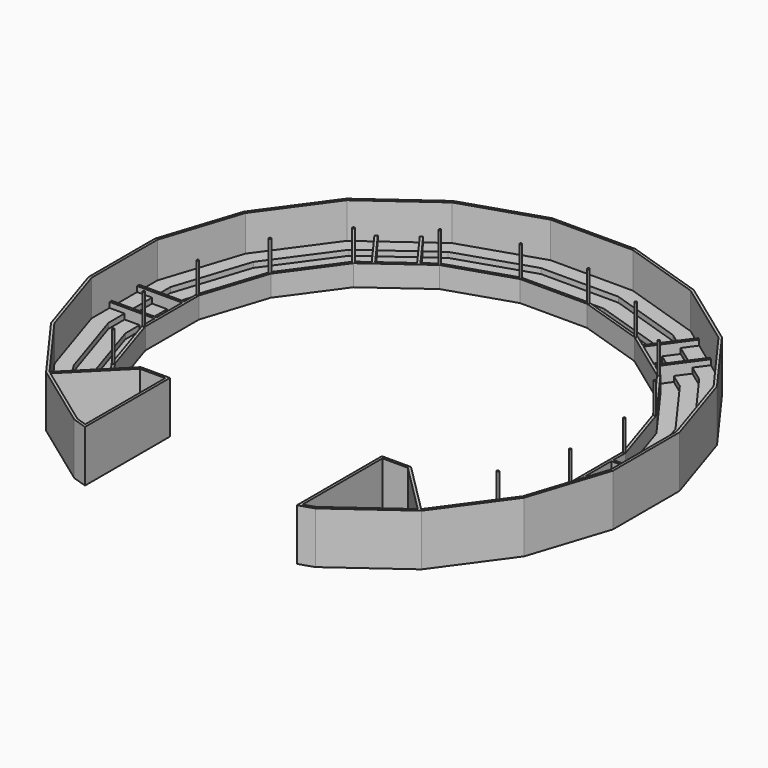
from build123d import *

# Parameters (mm, degrees)
F1_DEPTH = 2971.8
F2_DEPTH = 304.8
F0_W     = 863.6
F0_H     = 1828.8
F3_DEPTH = 609.6
F4_DEPTH = 914.4
F0_R     = 60.96
F5_DEPTH = 1219.2
F6_DEPTH = 2971.8


with BuildPart() as f1:
    # F0 (on Top) → F1 (new body)
    with BuildSketch(Plane.XY):
        Polygon((2389.6410818405, 15087.6), (-2389.6410818405, 15087.6), (-6935.0085268224, 13610.7205905095), (-8128.5036328315, 12743.5956390277), (-9655.127382741, 11634.4385604554), (-10801.5290181534, 10801.5290181534), (-13610.7205905095, 6935.0085268224), (-15087.6, 2389.6410818405), (-15087.6, 914.4), (-15087.6, 0), (-15087.6, -2389.6410818405), (-13610.7205905095, -6935.0085268224), (-10801.5290181534, -10801.5290181534), (-6935.0085268224, -13610.7205905095), (-6096, -13883.3309861815), (-6096, -7924.8), (-6096, -7772.4), (-7772.4, -7772.4), (-8728.5082974977, -8728.5082974977), (-8837.6146512164, -8837.6146512164), (-9455.8839889558, -9455.8839889558), (-10074.1533266953, -10074.1533266953), (-10692.4226644347, -10692.4226644347), (-13473.2385643428, -6864.9579356424), (-14935.2, -2365.503293135), (-14935.2, -1066.8), (-14935.2, -914.4), (-14935.2, 914.4), (-14935.2, 1066.8), (-14935.2, 2365.503293135), (-13473.2385643428, 6864.9579356424), (-10692.4226644347, 10692.4226644347), (-9688.8431002343, 11421.5658980633), (-9565.5489102916, 11511.1443705127), (-8038.9251603821, 12620.301449085), (-7915.6309704393, 12709.8799215343), (-6864.9579356424, 13473.2385643428), (-2365.503293135, 14935.2), (2365.503293135, 14935.2), (6864.9579356424, 13473.2385643428), (7915.6309704393, 12709.8799215343), (8038.9251603821, 12620.301449085), (9518.455439695, 11545.3597796925), (9641.7496296377, 11455.7813072431), (10692.4226644347, 10692.4226644347), (13473.2385643428, 6864.9579356424), (14935.2, 2365.503293135), (14935.2, 1066.8), (14935.2, 914.4), (14935.2, -914.4), (14935.2, -1066.8), (14935.2, -2365.503293135), (13473.2385643428, -6864.9579356424), (10692.4226644347, -10692.4226644347), (10074.1533266953, -10074.1533266953), (9455.8839889558, -9455.8839889558), (8837.6146512164, -8837.6146512164), (8728.5082974977, -8728.5082974977), (7772.4, -7772.4), (6705.6, -7772.4), (6096, -7772.4), (6096, -13883.3309861815), (6935.0085268224, -13610.7205905095), (10801.5290181534, -10801.5290181534), (13610.7205905095, -6935.0085268224), (15087.6, -2389.6410818405), (15087.6, -914.4), (15087.6, 914.4), (15087.6, 2389.6410818405), (13610.7205905095, 6935.0085268224), (10801.5290181534, 10801.5290181534), (6935.0085268224, 13610.7205905095), align=None)
        Polygon((-6864.9579356424, -13473.2385643428), (-10567.5915969054, -10783.117743811), (-7709.2738530943, -7924.8), (-6248.4, -7924.8), (-6248.4, -13673.5703815017), align=None, mode=Mode.SUBTRACT)
        Polygon((7709.2738530943, -7924.8), (10567.5915969054, -10783.117743811), (6864.9579356424, -13473.2385643428), (6248.4, -13673.5703815017), (6248.4, -7924.8), align=None, mode=Mode.SUBTRACT)
    extrude(amount=F1_DEPTH)


with BuildPart() as f2:
    # F0 (on Top) → F2 (new body)
    with BuildSketch(Plane.XY):
        Polygon((-9455.8839889558, -9455.8839889558), (-8837.6146512164, -8837.6146512164), (-11136.0441195078, -5674.097885582), (-12344.4, -1955.1608851422), (-12344.4, -1066.8), (-13208, -1066.8), (-13208, -2091.9416878065), (-11915.1089344528, -6071.0512356021), align=None)
    extrude(amount=F2_DEPTH)

    # F0 (on Top) → F3, piece 2 (join)
    with BuildSketch(Plane.XY):
        Polygon((-10074.1533266953, -10074.1533266953), (-9455.8839889558, -9455.8839889558), (-11915.1089344528, -6071.0512356021), (-13208, -2091.9416878065), (-13208, -1066.8), (-14071.6, -1066.8), (-14071.6, -2228.7224904707), (-12694.1737493978, -6468.0045856223), align=None)
    extrude(amount=F3_DEPTH)

    # F0 (on Top) → F4 (join)
    with BuildSketch(Plane.XY):
        Polygon((-10692.4226644347, -10692.4226644347), (-10074.1533266953, -10074.1533266953), (-12694.1737493978, -6468.0045856223), (-14071.6, -2228.7224904707), (-14071.6, -1066.8), (-14935.2, -1066.8), (-14935.2, -2365.503293135), (-13473.2385643428, -6864.9579356424), align=None)
    extrude(amount=F4_DEPTH)



with BuildPart() as f2b:
    # F0 (on Top) → F2, piece 2 (new body)
    with BuildSketch(Plane.XY):
        Polygon((-13208, 2091.9416878065), (-13208, 1066.8), (-12344.4, 1066.8), (-12344.4, 1955.1608851422), (-11136.0441195078, 5674.097885582), (-8837.6146512164, 8837.6146512164), (-8166.009068595, 9325.5646690367), (-8673.6204124748, 10024.2317453789), (-9455.8839889558, 9455.8839889558), (-11915.1089344528, 6071.0512356021), align=None)
    extrude(amount=F2_DEPTH)

    # F0 (on Top) → F3 (join)
    with BuildSketch(Plane.XY):
        Polygon((-14071.6, 2228.7224904707), (-14071.6, 1066.8), (-13208, 1066.8), (-13208, 2091.9416878065), (-11915.1089344528, 6071.0512356021), (-9455.8839889558, 9455.8839889558), (-8673.6204124748, 10024.2317453789), (-9181.2317563546, 10722.8988217211), (-10074.1533266953, 10074.1533266953), (-12694.1737493978, 6468.0045856223), align=None)
    extrude(amount=F3_DEPTH)

    # F0 (on Top) → F4, piece 2 (join)
    with BuildSketch(Plane.XY):
        Polygon((-14935.2, 2365.503293135), (-14935.2, 1066.8), (-14071.6, 1066.8), (-14071.6, 2228.7224904707), (-12694.1737493978, 6468.0045856223), (-10074.1533266953, 10074.1533266953), (-9181.2317563546, 10722.8988217211), (-9688.8431002343, 11421.5658980633), (-10692.4226644347, 10692.4226644347), (-13473.2385643428, 6864.9579356424), align=None)
    extrude(amount=F4_DEPTH)


with BuildPart() as f2c:
    # F0 (on Top) → F2, piece 3 (new body)
    with BuildSketch(Plane.XY):
        Polygon((11136.0441195078, -5674.097885582), (8837.6146512164, -8837.6146512164), (9455.8839889558, -9455.8839889558), (11915.1089344528, -6071.0512356021), (13208, -2091.9416878065), (13208, -1066.8), (12344.4, -1066.8), (12344.4, -1955.1608851422), align=None)
    extrude(amount=F2_DEPTH)

    # F0 (on Top) → F3, piece 5 (join)
    with BuildSketch(Plane.XY):
        Polygon((11915.1089344528, -6071.0512356021), (9455.8839889558, -9455.8839889558), (10074.1533266953, -10074.1533266953), (12694.1737493978, -6468.0045856223), (14071.6, -2228.7224904707), (14071.6, -1066.8), (13208, -1066.8), (13208, -2091.9416878065), align=None)
    extrude(amount=F3_DEPTH)

    # F0 (on Top) → F4, piece 5 (join)
    with BuildSketch(Plane.XY):
        Polygon((12694.1737493978, -6468.0045856223), (10074.1533266953, -10074.1533266953), (10692.4226644347, -10692.4226644347), (13473.2385643428, -6864.9579356424), (14935.2, -2365.503293135), (14935.2, -1066.8), (14071.6, -1066.8), (14071.6, -2228.7224904707), align=None)
    extrude(amount=F4_DEPTH)


with BuildPart() as f2d:
    # F0 (on Top) → F2, piece 4 (new body)
    with BuildSketch(Plane.XY):
        Polygon((12344.4, 1066.8), (13208, 1066.8), (13208, 2091.9416878065), (11915.1089344528, 6071.0512356021), (9455.8839889558, 9455.8839889558), (8626.5269418782, 10058.4471545587), (8118.9155979984, 9359.7800782165), (8837.6146512164, 8837.6146512164), (11136.0441195078, 5674.097885582), (12344.4, 1955.1608851422), align=None)
    extrude(amount=F2_DEPTH)

    # F0 (on Top) → F3, piece 4 (join)
    with BuildSketch(Plane.XY):
        Polygon((13208, 1066.8), (14071.6, 1066.8), (14071.6, 2228.7224904707), (12694.1737493978, 6468.0045856223), (10074.1533266953, 10074.1533266953), (9134.1382857579, 10757.1142309009), (8626.5269418782, 10058.4471545587), (9455.8839889558, 9455.8839889558), (11915.1089344528, 6071.0512356021), (13208, 2091.9416878065), align=None)
    extrude(amount=F3_DEPTH)

    # F0 (on Top) → F4, piece 4 (join)
    with BuildSketch(Plane.XY):
        Polygon((14071.6, 1066.8), (14935.2, 1066.8), (14935.2, 2365.503293135), (13473.2385643428, 6864.9579356424), (10692.4226644347, 10692.4226644347), (9641.7496296377, 11455.7813072431), (9134.1382857579, 10757.1142309009), (10074.1533266953, 10074.1533266953), (12694.1737493978, 6468.0045856223), (14071.6, 2228.7224904707), align=None)
    extrude(amount=F4_DEPTH)


with BuildPart() as f2e:
    # F0 (on Top) → F2, piece 5 (new body)
    with BuildSketch(Plane.XY):
        Polygon((-1955.1608851422, 12344.4), (0, 12344.4), (1955.1608851422, 12344.4), (5674.097885582, 11136.0441195078), (6392.7969388, 10613.8786925077), (6900.4082826798, 11312.5457688499), (6071.0512356021, 11915.1089344528), (2091.9416878065, 13208), (-2091.9416878065, 13208), (-6071.0512356021, 11915.1089344528), (-6900.4082826798, 11312.5457688499), (-6392.7969388, 10613.8786925077), (-5674.097885582, 11136.0441195078), align=None)
    extrude(amount=F2_DEPTH)

    # F0 (on Top) → F3, piece 3 (join)
    with BuildSketch(Plane.XY):
        Polygon((-7408.0196265596, 12011.2128451921), (-6900.4082826798, 11312.5457688499), (-6071.0512356021, 11915.1089344528), (-2091.9416878065, 13208), (2091.9416878065, 13208), (6071.0512356021, 11915.1089344528), (6900.4082826798, 11312.5457688499), (7408.0196265596, 12011.2128451921), (6468.0045856223, 12694.1737493978), (2228.7224904707, 14071.6), (-2228.7224904707, 14071.6), (-6468.0045856223, 12694.1737493978), align=None)
    extrude(amount=F3_DEPTH)

    # F0 (on Top) → F4, piece 3 (join)
    with BuildSketch(Plane.XY):
        Polygon((7408.0196265596, 12011.2128451921), (7915.6309704393, 12709.8799215343), (6864.9579356424, 13473.2385643428), (2365.503293135, 14935.2), (-2365.503293135, 14935.2), (-6864.9579356424, 13473.2385643428), (-7915.6309704393, 12709.8799215343), (-7408.0196265596, 12011.2128451921), (-6468.0045856223, 12694.1737493978), (-2228.7224904707, 14071.6), (2228.7224904707, 14071.6), (6468.0045856223, 12694.1737493978), align=None)
    extrude(amount=F4_DEPTH)


with BuildPart() as f2f:
    # F0 (on Top) → F2, piece 6 (new body)
    with BuildSketch(Plane.XY):
        with Locations((-12776.2, 0)):
            Rectangle(F0_W, F0_H)
    extrude(amount=F2_DEPTH)

    # F0 (on Top) → F3, piece 6 (join)
    with BuildSketch(Plane.XY):
        with Locations((-13639.8, 0)):
            Rectangle(F0_W, F0_H)
    extrude(amount=F3_DEPTH)

    # F0 (on Top) → F4, piece 6 (join)
    with BuildSketch(Plane.XY):
        with Locations((-14503.4, 0)):
            Rectangle(F0_W, F0_H)
    extrude(amount=F4_DEPTH)


with BuildPart() as f2g:
    # F0 (on Top) → F2, piece 7 (new body)
    with BuildSketch(Plane.XY):
        Polygon((-7023.7024726225, 11222.9672964006), (-8550.326222532, 10113.8102178283), (-8042.7148786523, 9415.1431414861), (-6516.0911287427, 10524.3002200584), align=None)
    extrude(amount=F2_DEPTH)

    # F0 (on Top) → F3, piece 7 (join)
    with BuildSketch(Plane.XY):
        Polygon((-7531.3138165023, 11921.6343727428), (-9057.9375664118, 10812.4772941705), (-8550.326222532, 10113.8102178283), (-7023.7024726225, 11222.9672964006), align=None)
    extrude(amount=F3_DEPTH)

    # F0 (on Top) → F4, piece 7 (join)
    with BuildSketch(Plane.XY):
        Polygon((-8038.9251603821, 12620.301449085), (-9565.5489102916, 11511.1443705127), (-9057.9375664118, 10812.4772941705), (-7531.3138165023, 11921.6343727428), align=None)
    extrude(amount=F4_DEPTH)


with BuildPart() as f2h:
    # F0 (on Top) → F2, piece 8 (new body)
    with BuildSketch(Plane.XY):
        Polygon((7995.6214080556, 9449.3585506659), (8503.2327519354, 10148.0256270081), (7023.7024726225, 11222.9672964006), (6516.0911287427, 10524.3002200584), align=None)
    extrude(amount=F2_DEPTH)

    # F0 (on Top) → F3, piece 8 (join)
    with BuildSketch(Plane.XY):
        Polygon((8503.2327519354, 10148.0256270081), (9010.8440958152, 10846.6927033503), (7531.3138165023, 11921.6343727428), (7023.7024726225, 11222.9672964006), align=None)
    extrude(amount=F3_DEPTH)

    # F0 (on Top) → F4, piece 8 (join)
    with BuildSketch(Plane.XY):
        Polygon((9010.8440958152, 10846.6927033503), (9518.455439695, 11545.3597796925), (8038.9251603821, 12620.301449085), (7531.3138165023, 11921.6343727428), align=None)
    extrude(amount=F4_DEPTH)


with BuildPart() as f2i:
    # F0 (on Top) → F2, piece 9 (new body)
    with BuildSketch(Plane.XY):
        with Locations((12776.2, 0)):
            Rectangle(F0_W, F0_H)
    extrude(amount=F2_DEPTH)

    # F0 (on Top) → F3, piece 9 (join)
    with BuildSketch(Plane.XY):
        with Locations((13639.8, 0)):
            Rectangle(F0_W, F0_H)
    extrude(amount=F3_DEPTH)

    # F0 (on Top) → F4, piece 9 (join)
    with BuildSketch(Plane.XY):
        with Locations((14503.4, 0)):
            Rectangle(F0_W, F0_H)
    extrude(amount=F4_DEPTH)


with BuildPart() as f2_1:
    add(f2.part)

    add(f2b.part)  # F5 merges F2b

    add(f2c.part)  # F5 merges F2c

    add(f2d.part)  # F5 merges F2d

    add(f2e.part)  # F5 merges F2e

    add(f2f.part)  # F5 merges F2f

    add(f2g.part)  # F5 merges F2g

    add(f2h.part)  # F5 merges F2h

    add(f2i.part)  # F5 merges F2i
    # F0 (on Top) → F5 (join)
    with BuildSketch(Plane.XY):
        Polygon((-8837.6146512164, -8837.6146512164), (-8728.5082974977, -8728.5082974977), (-10998.562093341, -5604.047294402), (-12192, -1931.0230964367), (-12192, -914.4), (-12192, 914.4), (-12192, 1931.0230964367), (-10998.562093341, 5604.047294402), (-8728.5082974977, 8728.5082974977), (-7953.1364062029, 9291.8489515433), (-6426.5126562934, 10401.0060301156), (-5604.047294402, 10998.562093341), (-1931.0230964367, 12192), (0, 12192), (0, 12344.4), (-1955.1608851422, 12344.4), (-5674.097885582, 11136.0441195078), (-6392.7969388, 10613.8786925077), (-6900.4082826798, 11312.5457688499), (-7408.0196265596, 12011.2128451921), (-7915.6309704393, 12709.8799215343), (-8038.9251603821, 12620.301449085), (-7531.3138165023, 11921.6343727428), (-7023.7024726225, 11222.9672964006), (-6516.0911287427, 10524.3002200584), (-8042.7148786523, 9415.1431414861), (-8550.326222532, 10113.8102178283), (-9057.9375664118, 10812.4772941705), (-9565.5489102916, 11511.1443705127), (-9688.8431002343, 11421.5658980633), (-9181.2317563546, 10722.8988217211), (-8673.6204124748, 10024.2317453789), (-8166.009068595, 9325.5646690367), (-8837.6146512164, 8837.6146512164), (-11136.0441195078, 5674.097885582), (-12344.4, 1955.1608851422), (-12344.4, 1066.8), (-13208, 1066.8), (-14071.6, 1066.8), (-14935.2, 1066.8), (-14935.2, 914.4), (-14071.6, 914.4), (-13208, 914.4), (-12344.4, 914.4), (-12344.4, -914.4), (-13208, -914.4), (-14071.6, -914.4), (-14935.2, -914.4), (-14935.2, -1066.8), (-14071.6, -1066.8), (-13208, -1066.8), (-12344.4, -1066.8), (-12344.4, -1955.1608851422), (-11136.0441195078, -5674.097885582), align=None)
        with Locations((-11067.3031064244, -5639.072589992)):
            Circle(F0_R, mode=Mode.SUBTRACT)
        with Locations((-12268.2, -1943.0919907895)):
            Circle(F0_R, mode=Mode.SUBTRACT)
        with Locations((-12268.2, 1943.0919907895)):
            Circle(F0_R, mode=Mode.SUBTRACT)
        with Locations((-11067.3031064244, 5639.072589992)):
            Circle(F0_R, mode=Mode.SUBTRACT)
        with Locations((-8783.0614743571, 8783.0614743571)):
            Circle(F0_R, mode=Mode.SUBTRACT)
        with Locations((-5639.072589992, 11067.3031064244)):
            Circle(F0_R, mode=Mode.SUBTRACT)
        with Locations((-1943.0919907895, 12268.2)):
            Circle(F0_R, mode=Mode.SUBTRACT)
        Polygon((10998.562093341, -5604.047294402), (8728.5082974977, -8728.5082974977), (8837.6146512164, -8837.6146512164), (11136.0441195078, -5674.097885582), (12344.4, -1955.1608851422), (12344.4, -1066.8), (13208, -1066.8), (14071.6, -1066.8), (14935.2, -1066.8), (14935.2, -914.4), (14071.6, -914.4), (13208, -914.4), (12344.4, -914.4), (12344.4, 914.4), (13208, 914.4), (14071.6, 914.4), (14935.2, 914.4), (14935.2, 1066.8), (14071.6, 1066.8), (13208, 1066.8), (12344.4, 1066.8), (12344.4, 1955.1608851422), (11136.0441195078, 5674.097885582), (8837.6146512164, 8837.6146512164), (8118.9155979984, 9359.7800782165), (8626.5269418782, 10058.4471545587), (9134.1382857579, 10757.1142309009), (9641.7496296377, 11455.7813072431), (9518.455439695, 11545.3597796925), (9010.8440958152, 10846.6927033503), (8503.2327519354, 10148.0256270081), (7995.6214080556, 9449.3585506659), (6516.0911287427, 10524.3002200584), (7023.7024726225, 11222.9672964006), (7531.3138165023, 11921.6343727428), (8038.9251603821, 12620.301449085), (7915.6309704393, 12709.8799215343), (7408.0196265596, 12011.2128451921), (6900.4082826798, 11312.5457688499), (6392.7969388, 10613.8786925077), (5674.097885582, 11136.0441195078), (1955.1608851422, 12344.4), (0, 12344.4), (0, 12192), (1931.0230964367, 12192), (5604.047294402, 10998.562093341), (6426.5126562934, 10401.0060301156), (7906.0429356063, 9326.0643607231), (8728.5082974977, 8728.5082974977), (10998.562093341, 5604.047294402), (12192, 1931.0230964367), (12192, 914.4), (12192, -914.4), (12192, -1931.0230964367), align=None)
        with Locations((11067.3031064244, -5639.072589992)):
            Circle(F0_R, mode=Mode.SUBTRACT)
        with Locations((12268.2, -1943.0919907895)):
            Circle(F0_R, mode=Mode.SUBTRACT)
        with Locations((12268.2, 1943.0919907895)):
            Circle(F0_R, mode=Mode.SUBTRACT)
        with Locations((11067.3031064244, 5639.072589992)):
            Circle(F0_R, mode=Mode.SUBTRACT)
        with Locations((5639.072589992, 11067.3031064244)):
            Circle(F0_R, mode=Mode.SUBTRACT)
        with Locations((1943.0919907895, 12268.2)):
            Circle(F0_R, mode=Mode.SUBTRACT)
        with Locations((8783.0614743571, 8783.0614743571)):
            Circle(F0_R, mode=Mode.SUBTRACT)
    extrude(amount=F5_DEPTH)

    # F0 (on Top) → F6 (join)
    with BuildSketch(Plane.XY):
        with Locations((-11067.3031064244, -5639.072589992)):
            Circle(F0_R)
        with Locations((-12268.2, -1943.0919907895)):
            Circle(F0_R)
        with Locations((-12268.2, 1943.0919907895)):
            Circle(F0_R)
        with Locations((-11067.3031064244, 5639.072589992)):
            Circle(F0_R)
        with Locations((-8783.0614743571, 8783.0614743571)):
            Circle(F0_R)
        with Locations((-5639.072589992, 11067.3031064244)):
            Circle(F0_R)
        with Locations((-1943.0919907895, 12268.2)):
            Circle(F0_R)
        with Locations((1943.0919907895, 12268.2)):
            Circle(F0_R)
        with Locations((5639.072589992, 11067.3031064244)):
            Circle(F0_R)
        with Locations((8783.0614743571, 8783.0614743571)):
            Circle(F0_R)
        with Locations((11067.3031064244, 5639.072589992)):
            Circle(F0_R)
        with Locations((12268.2, 1943.0919907895)):
            Circle(F0_R)
        with Locations((12268.2, -1943.0919907895)):
            Circle(F0_R)
        with Locations((11067.3031064244, -5639.072589992)):
            Circle(F0_R)
    extrude(amount=F6_DEPTH)


solid = Compound([f1.part, f2_1.part])
